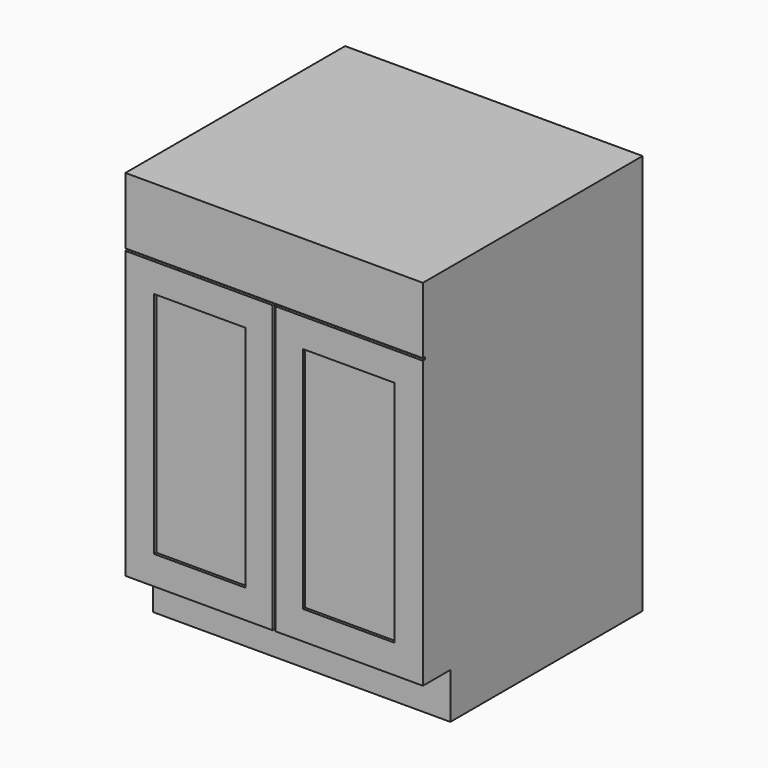
from build123d import *

# Parameters (mm, degrees)
F0_W     = 3.175
F0_H     = 635
F0_W_2   = 327.025
F0_W_3   = 203.2
F0_H_2   = 508
F0_W_4   = 330.2
F0_H_3   = 147.32
F1_DEPTH = 609.6
F2_DEPTH = 6.35
F3_DEPTH = 76.2


with BuildPart() as f1:
    # F0 (on Front) → F1 (new body)
    with BuildSketch(Plane.XZ):
        Polygon((227.9072425127, -101.6), (227.9072425127, 0), (224.7322425127, 0), (-102.2927574873, 0), (-102.2927574873, -101.6), align=None)
        with Locations((226.3197425127, 317.5)):
            Rectangle(F0_W, F0_H)
        Polygon((231.0822425127, 0), (227.9072425127, 0), (227.9072425127, -101.6), (558.1072425127, -101.6), (558.1072425127, 0), align=None)
        with Locations((229.4947425127, 317.5)):
            Rectangle(F0_W, F0_H)
        with Locations((61.2197425127, 317.5)):
            Rectangle(F0_W_2, F0_H)
        with Locations((62.8072425127, 317.5)):
            Rectangle(F0_W_3, F0_H_2, mode=Mode.SUBTRACT)
        Polygon((224.7322425127, 635), (227.9072425127, 635), (227.9072425127, 640.08), (-102.2927574873, 640.08), (-102.2927574873, 635), align=None)
        Polygon((227.9072425127, 640.08), (227.9072425127, 635), (231.0822425127, 635), (558.1072425127, 635), (558.1072425127, 640.08), align=None)
        with Locations((394.5947425127, 317.5)):
            Rectangle(F0_W_2, F0_H)
        with Locations((393.0072425127, 317.5)):
            Rectangle(F0_W_3, F0_H_2, mode=Mode.SUBTRACT)
        with Locations((62.8072425127, 713.74)):
            Rectangle(F0_W_4, F0_H_3)
        with Locations((393.0072425127, 713.74)):
            Rectangle(F0_W_4, F0_H_3)
        with Locations((62.8072425127, 317.5)):
            Rectangle(F0_W_3, F0_H_2)
        with Locations((393.0072425127, 317.5)):
            Rectangle(F0_W_3, F0_H_2)
    extrude(amount=-F1_DEPTH)

    # F0 (on Front) → F2 (cut)
    with BuildSketch(Plane.XZ):
        with Locations((226.3197425127, 317.5)):
            Rectangle(F0_W, F0_H)
        with Locations((229.4947425127, 317.5)):
            Rectangle(F0_W, F0_H)
        Polygon((224.7322425127, 635), (227.9072425127, 635), (227.9072425127, 640.08), (-102.2927574873, 640.08), (-102.2927574873, 635), align=None)
        Polygon((227.9072425127, 640.08), (227.9072425127, 635), (231.0822425127, 635), (558.1072425127, 635), (558.1072425127, 640.08), align=None)
        with Locations((62.8072425127, 317.5)):
            Rectangle(F0_W_3, F0_H_2)
        with Locations((393.0072425127, 317.5)):
            Rectangle(F0_W_3, F0_H_2)
    extrude(amount=-F2_DEPTH, mode=Mode.SUBTRACT)

    # F0 (on Front) → F3 (cut)
    with BuildSketch(Plane.XZ):
        Polygon((227.9072425127, -101.6), (227.9072425127, 0), (224.7322425127, 0), (-102.2927574873, 0), (-102.2927574873, -101.6), align=None)
        Polygon((231.0822425127, 0), (227.9072425127, 0), (227.9072425127, -101.6), (558.1072425127, -101.6), (558.1072425127, 0), align=None)
    extrude(amount=-F3_DEPTH, mode=Mode.SUBTRACT)


solid = f1.part
